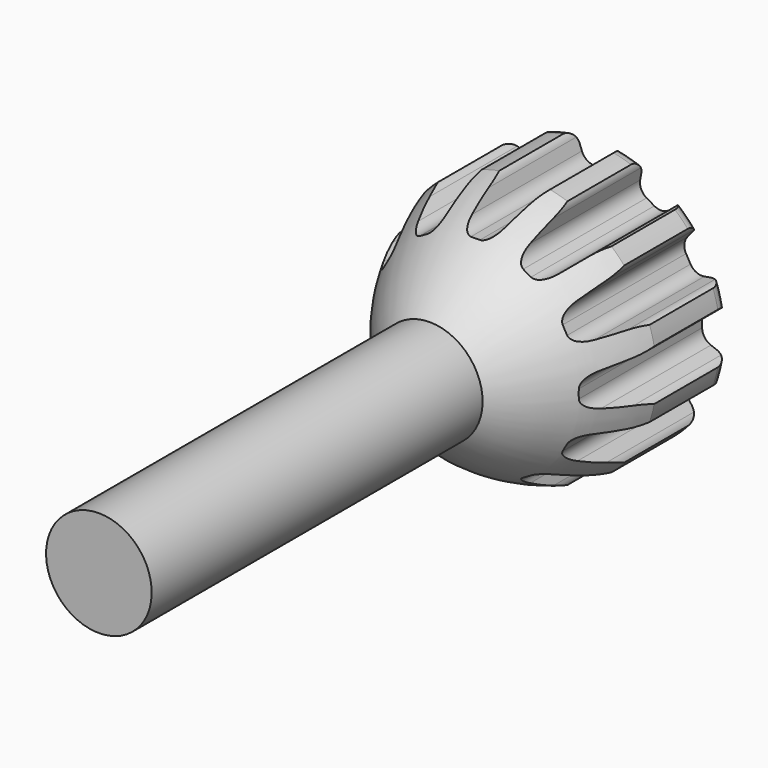
from build123d import *

# Parameters (mm, degrees)
F0_W            = 156.6659212112
F0_H            = 20
F3_DEPTH        = 201.6956955194
F3_COPIES_COUNT = 12


# Not quite as in the source:
# - a feature of the source that left no trace in its solid (it failed there, or was rolled back) is left out
# - a pattern or mirror of a feature is missing from the dataset's text; its kind, count and spacing are read off the source's solid


with BuildPart() as f1:
    # F0 (on Right) → F1 (revolve)
    with BuildSketch(Plane.YZ):
        Rectangle(F0_W, F0_H)
        with BuildLine():
            Line((78.3329606056, 10), (78.3329606056, -10))
            Line((78.3329606056, -10), (144.0980745316, -10))
            Line((144.0980745316, -10), (144.0980745316, -9.4412732124))
            ThreePointArc((144.0980745316, -9.4412732124), (145.5625406256, -5.9057393065), (149.0980745316, -4.4412732124))
            Line((149.0980745316, -4.4412732124), (153.3329606056, -4.4412732124))
            ThreePointArc((153.3329606056, -4.4412732124), (156.8684945116, -2.9768071184), (158.3329606056, 0.5587267876))
            Line((158.3329606056, 0.5587267876), (158.3329606056, 35))
            ThreePointArc((158.3329606056, 35), (156.8684945116, 38.5355339059), (153.3329606056, 40))
            Line((153.3329606056, 40), (123.232871294, 40))
            ThreePointArc((123.232871294, 40), (98.5802664321, 28.2966255541), (78.3329606056, 10))
        make_face()
    revolve(axis=Axis((0, 0, -10), (0, -1, 0)))

    # F2 (on Front) → F3 (cut)
    with BuildSketch(Plane.XZ):
        with BuildLine():
            Line((-1.698962309, 29.1487361115), (0, 29.1487361115))
            Line((0, 29.1487361115), (1.698962309, 29.1487361115))
            ThreePointArc((1.698962309, 29.1487361115), (4.5668444907, 30.05297589), (6.3974254129, 32.4386353948))
            Line((6.3974254129, 32.4386353948), (8, 36.8416728859))
            ThreePointArc((8, 36.8416728859), (12.2277513661, 40.1093659035), (16.9930875315, 37.6920801319))
            Line((16.9930875315, 37.6920801319), (17.4989907375, 37.9844652277))
            Line((17.4989907375, 37.9844652277), (0, 51.1487361115))
            Line((0, 51.1487361115), (-17.4989907375, 37.9844652277))
            Line((-17.4989907375, 37.9844652277), (-16.9930875315, 37.6920801319))
            ThreePointArc((-16.9930875315, 37.6920801319), (-12.2277513661, 40.1093659035), (-8, 36.8416728859))
            Line((-8, 36.8416728859), (-6.3974254129, 32.4386353948))
            ThreePointArc((-6.3974254129, 32.4386353948), (-4.5668444907, 30.05297589), (-1.698962309, 29.1487361115))
        make_face()
    f3 = extrude(amount=-F3_DEPTH, mode=Mode.SUBTRACT)

    # F3_copies: F3 ×12 about axis
    f3_copies_axis = Axis((0, 0, -10.000002), (0, 1, 0))
    for i in range(1, F3_COPIES_COUNT):
        add(f3.rotate(f3_copies_axis, i * 360 / F3_COPIES_COUNT), mode=Mode.SUBTRACT)


solid = f1.part
